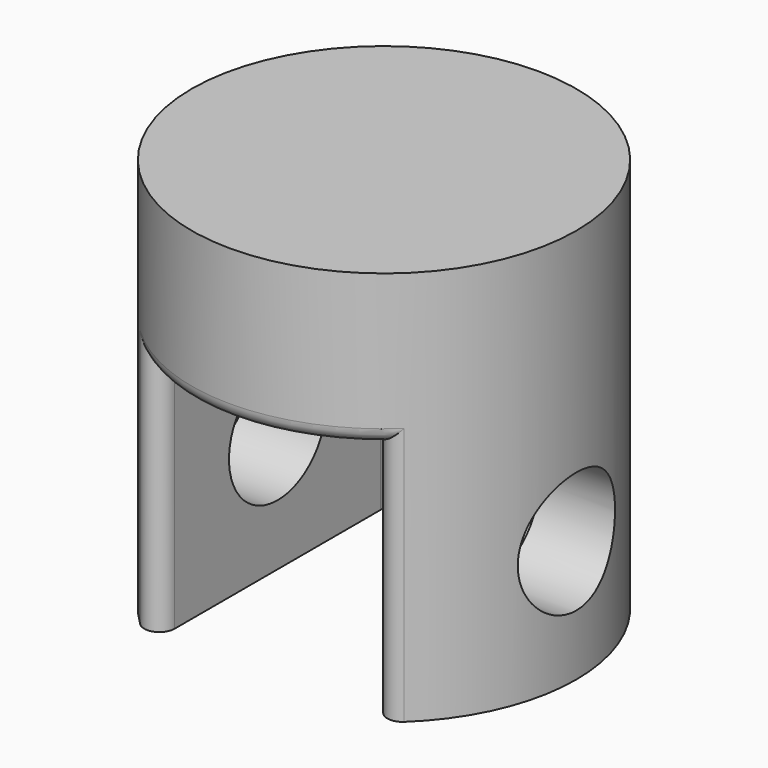
from build123d import *

# Parameters (mm, degrees)
F0_R         = 12.65
F1_DEPTH     = 26
F2_W         = 14
F2_H         = 29.3698692877
F3_DEPTH     = 16
F4_T1_DEPTH  = 21.3868200642
F4_T6_ANGLE  = 89.8472397972
F4_T12_ANGLE = 89.8472397972
F4_T19_DEPTH = 26.7736401284
F4_T23_ANGLE = 89.8472397972
F4_T30_ANGLE = 89.8472397972
F4_T34_DEPTH = 26.7736401284
F4_T41_ANGLE = 89.8472397972
F4_T45_DEPTH = 26.7736401284
F4_T52_DEPTH = 26.7736401284
F4_T56_ANGLE = 89.8472397972
F5_R         = 4
F6_DEPTH     = 16.2


# Not quite as in the source:
# - a fillet or chamfer that OpenCascade refuses, or shapes differently, is made with other operations: its cross-section is extruded or revolved along the edge and cut away or added


with BuildPart() as f1:
    # F0 (on Top) → F1 (new body)
    with BuildSketch(Plane.XY):
        Circle(F0_R)
    extrude(amount=F1_DEPTH)

    # F2 (on Top) → F3 (cut)
    with BuildSketch(Plane.XY):
        Rectangle(F2_W, F2_H)
    extrude(amount=F3_DEPTH, mode=Mode.SUBTRACT)

    # F4: fillet of radius 1 on 6 edges, made by hand

    # F4_s2 → F4_t1 (cut)
    with BuildSketch(Plane.XY.offset(-5.3868200642)):
        with BuildLine():
            ThreePointArc((8.686695279, 9.1958591295), (7.6042066694, 9.3872533539), (7, 8.4689137438))
            Line((7, 8.4689137438), (7, 10.5367215015))
            ThreePointArc((7, 10.5367215015), (7.8719489435, 9.9022684185), (8.686695279, 9.1958591295))
        make_face()
        with BuildLine():
            ThreePointArc((8.686695279, -9.1958591295), (7.6042066694, -9.3872533539), (7, -8.4689137438))
            Line((7, -8.4689137438), (7, -10.5367215015))
            ThreePointArc((7, -10.5367215015), (7.8719489435, -9.9022684185), (8.686695279, -9.1958591295))
        make_face()
        with BuildLine():
            ThreePointArc((-8.686695279, 9.1958591295), (-7.6042066694, 9.3872533539), (-7, 8.4689137438))
            Line((-7, 8.4689137438), (-7, 10.5367215015))
            ThreePointArc((-7, 10.5367215015), (-7.8719489435, 9.9022684185), (-8.686695279, 9.1958591295))
        make_face()
        with BuildLine():
            ThreePointArc((-8.686695279, -9.1958591295), (-7.6042066694, -9.3872533539), (-7, -8.4689137438))
            Line((-7, -8.4689137438), (-7, -10.5367215015))
            ThreePointArc((-7, -10.5367215015), (-7.8719489435, -9.9022684185), (-8.686695279, -9.1958591295))
        make_face()
    extrude(amount=F4_T1_DEPTH, mode=Mode.SUBTRACT)


with BuildPart() as f4_tool4:
    # F4_s5 → F4_t6 (revolve)
    with BuildSketch(Plane(origin=(0, 0, 0), x_dir=(0, 0, 1), z_dir=(-0.7080487855, -0.7061635202, 0))):
        with BuildLine():
            ThreePointArc((17, 12.65), (16.2928932188, 12.3571067812), (16, 11.65))
            Line((16, 11.65), (16, 12.65))
            Line((16, 12.65), (17, 12.65))
        make_face()
    revolve(axis=Axis((0, 0, 16), (0, 0, -1)), revolution_arc=F4_T6_ANGLE)

    split(bisect_by=Plane.YZ.offset(7), keep=Keep.BOTTOM)

    split(bisect_by=Plane.YZ.offset(-7), keep=Keep.TOP)


with BuildPart() as f1_1:
    add(f1.part)

    # F4_t3: cut F4_tool4
    add(f4_tool4.part, mode=Mode.SUBTRACT)


with BuildPart() as f4_tool10:
    # F4_s11 → F4_t12 (revolve)
    with BuildSketch(Plane(origin=(0, 0, 0), x_dir=(0, 0, 1), z_dir=(0.7080487855, 0.7061635202, 0))):
        with BuildLine():
            ThreePointArc((17, 12.65), (16.2928932188, 12.3571067812), (16, 11.65))
            Line((16, 11.65), (16, 12.65))
            Line((16, 12.65), (17, 12.65))
        make_face()
    revolve(axis=Axis((0, 0, 16), (0, 0, -1)), revolution_arc=F4_T12_ANGLE)

    split(bisect_by=Plane.YZ.offset(7), keep=Keep.BOTTOM)

    split(bisect_by=Plane.YZ.offset(-7), keep=Keep.TOP)


with BuildPart() as f1_2:
    add(f1_1.part)

    # F4_t9: cut F4_tool10
    add(f4_tool10.part, mode=Mode.SUBTRACT)


with BuildPart() as f4_tool17:
    # F4_s18 → F4_t19 (new body)
    with BuildSketch(Plane.XY.offset(21.3868200642)):
        with BuildLine():
            ThreePointArc((8.686695279, 9.1958591295), (7.6042066694, 9.3872533539), (7, 8.4689137438))
            Line((7, 8.4689137438), (7, 10.5367215015))
            ThreePointArc((7, 10.5367215015), (7.8719489435, 9.9022684185), (8.686695279, 9.1958591295))
        make_face()
    extrude(amount=-F4_T19_DEPTH)

    split(bisect_by=Plane.XY.offset(16), keep=Keep.TOP)


with BuildPart() as f4_tool21:
    # F4_s22 → F4_t23 (revolve)
    with BuildSketch(Plane(origin=(0, 0, 0), x_dir=(0, 0, 1), z_dir=(-0.7080487855, -0.7061635202, 0))):
        with BuildLine():
            ThreePointArc((17, 12.65), (16.2928932188, 12.3571067812), (16, 11.65))
            Line((16, 11.65), (16, 12.65))
            Line((16, 12.65), (17, 12.65))
        make_face()
    revolve(axis=Axis((0, 0, 16), (0, 0, -1)), revolution_arc=F4_T23_ANGLE)

    split(bisect_by=Plane.YZ.offset(7), keep=Keep.TOP)


with BuildPart() as f4_tool17_1:
    add(f4_tool17.part)

    # F4_t25: intersect F4_tool21
    add(f4_tool21.part, mode=Mode.INTERSECT)


with BuildPart() as f1_3:
    add(f1_2.part)

    # F4_t15: cut F4_tool17
    add(f4_tool17_1.part, mode=Mode.SUBTRACT)


with BuildPart() as f4_tool28:
    # F4_s29 → F4_t30 (revolve)
    with BuildSketch(Plane(origin=(0, 0, 0), x_dir=(0, 0, 1), z_dir=(0.7080487855, 0.7061635202, 0))):
        with BuildLine():
            ThreePointArc((17, 12.65), (16.2928932188, 12.3571067812), (16, 11.65))
            Line((16, 11.65), (16, 12.65))
            Line((16, 12.65), (17, 12.65))
        make_face()
    revolve(axis=Axis((0, 0, 16), (0, 0, -1)), revolution_arc=F4_T30_ANGLE)

    split(bisect_by=Plane.YZ.offset(7), keep=Keep.TOP)


with BuildPart() as f4_tool32:
    # F4_s33 → F4_t34 (new body)
    with BuildSketch(Plane.XY.offset(21.3868200642)):
        with BuildLine():
            ThreePointArc((8.686695279, -9.1958591295), (7.6042066694, -9.3872533539), (7, -8.4689137438))
            Line((7, -8.4689137438), (7, -10.5367215015))
            ThreePointArc((7, -10.5367215015), (7.8719489435, -9.9022684185), (8.686695279, -9.1958591295))
        make_face()
    extrude(amount=-F4_T34_DEPTH)

    split(bisect_by=Plane.XY.offset(16), keep=Keep.TOP)


with BuildPart() as f4_tool28_1:
    add(f4_tool28.part)

    # F4_t36: intersect F4_tool32
    add(f4_tool32.part, mode=Mode.INTERSECT)


with BuildPart() as f1_4:
    add(f1_3.part)

    # F4_t26: cut F4_tool28
    add(f4_tool28_1.part, mode=Mode.SUBTRACT)


with BuildPart() as f4_tool39:
    # F4_s40 → F4_t41 (revolve)
    with BuildSketch(Plane(origin=(0, 0, 0), x_dir=(0, 0, 1), z_dir=(-0.7080487855, -0.7061635202, 0))):
        with BuildLine():
            ThreePointArc((17, 12.65), (16.2928932188, 12.3571067812), (16, 11.65))
            Line((16, 11.65), (16, 12.65))
            Line((16, 12.65), (17, 12.65))
        make_face()
    revolve(axis=Axis((0, 0, 16), (0, 0, -1)), revolution_arc=F4_T41_ANGLE)

    split(bisect_by=Plane.YZ.offset(-7), keep=Keep.BOTTOM)


with BuildPart() as f4_tool43:
    # F4_s44 → F4_t45 (new body)
    with BuildSketch(Plane.XY.offset(21.3868200642)):
        with BuildLine():
            ThreePointArc((-8.686695279, 9.1958591295), (-7.6042066694, 9.3872533539), (-7, 8.4689137438))
            Line((-7, 8.4689137438), (-7, 10.5367215015))
            ThreePointArc((-7, 10.5367215015), (-7.8719489435, 9.9022684185), (-8.686695279, 9.1958591295))
        make_face()
    extrude(amount=-F4_T45_DEPTH)

    split(bisect_by=Plane.XY.offset(16), keep=Keep.TOP)


with BuildPart() as f4_tool39_1:
    add(f4_tool39.part)

    # F4_t47: intersect F4_tool43
    add(f4_tool43.part, mode=Mode.INTERSECT)


with BuildPart() as f1_5:
    add(f1_4.part)

    # F4_t37: cut F4_tool39
    add(f4_tool39_1.part, mode=Mode.SUBTRACT)


with BuildPart() as f4_tool50:
    # F4_s51 → F4_t52 (new body)
    with BuildSketch(Plane.XY.offset(21.3868200642)):
        with BuildLine():
            ThreePointArc((-8.686695279, -9.1958591295), (-7.6042066694, -9.3872533539), (-7, -8.4689137438))
            Line((-7, -8.4689137438), (-7, -10.5367215015))
            ThreePointArc((-7, -10.5367215015), (-7.8719489435, -9.9022684185), (-8.686695279, -9.1958591295))
        make_face()
    extrude(amount=-F4_T52_DEPTH)

    split(bisect_by=Plane.XY.offset(16), keep=Keep.TOP)


with BuildPart() as f4_tool54:
    # F4_s55 → F4_t56 (revolve)
    with BuildSketch(Plane(origin=(0, 0, 0), x_dir=(0, 0, 1), z_dir=(0.7080487855, 0.7061635202, 0))):
        with BuildLine():
            ThreePointArc((17, 12.65), (16.2928932188, 12.3571067812), (16, 11.65))
            Line((16, 11.65), (16, 12.65))
            Line((16, 12.65), (17, 12.65))
        make_face()
    revolve(axis=Axis((0, 0, 16), (0, 0, -1)), revolution_arc=F4_T56_ANGLE)

    split(bisect_by=Plane.YZ.offset(-7), keep=Keep.BOTTOM)


with BuildPart() as f4_tool50_1:
    add(f4_tool50.part)

    # F4_t58: intersect F4_tool54
    add(f4_tool54.part, mode=Mode.INTERSECT)


with BuildPart() as f1_6:
    add(f1_5.part)

    # F4_t48: cut F4_tool50
    add(f4_tool50_1.part, mode=Mode.SUBTRACT)

    # F5 (on Right) → F6 (cut, symmetric)
    with BuildSketch(Plane.YZ):
        with Locations((0, 8)):
            Circle(F5_R)
    extrude(amount=F6_DEPTH, both=True, mode=Mode.SUBTRACT)


solid = f1_6.part
